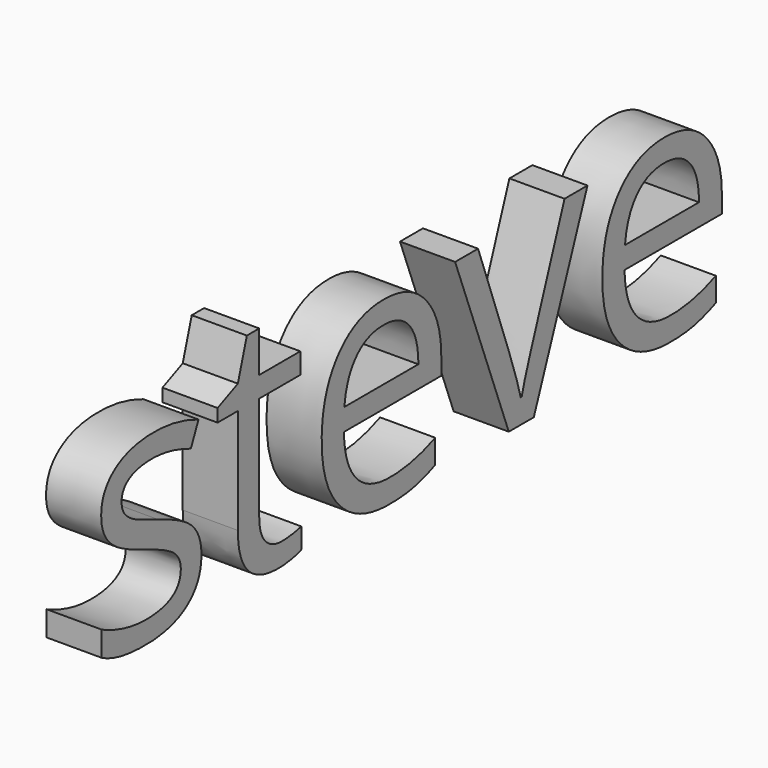
from build123d import *

# Parameters (mm, degrees)
F0_TEXT_SIZE = 38.0556487168
F1_DEPTH     = 6.35


# Not quite as in the source:
# - Text() gives the source's letters only with a copy of the font that has no kerning and outlines rounded to 1/6400 em; it was checked with that copy


with BuildPart() as f1:
    # F0 (on Right) → F1 (new body)
    with BuildSketch(Plane.YZ):
        with Locations((-55.3675703704, 21.1904961616)):
            Text('steve', F0_TEXT_SIZE, font='Open Sans', text_align=(TextAlign.LEFT, TextAlign.BOTTOM))
    extrude(amount=F1_DEPTH)


solid = f1.part
